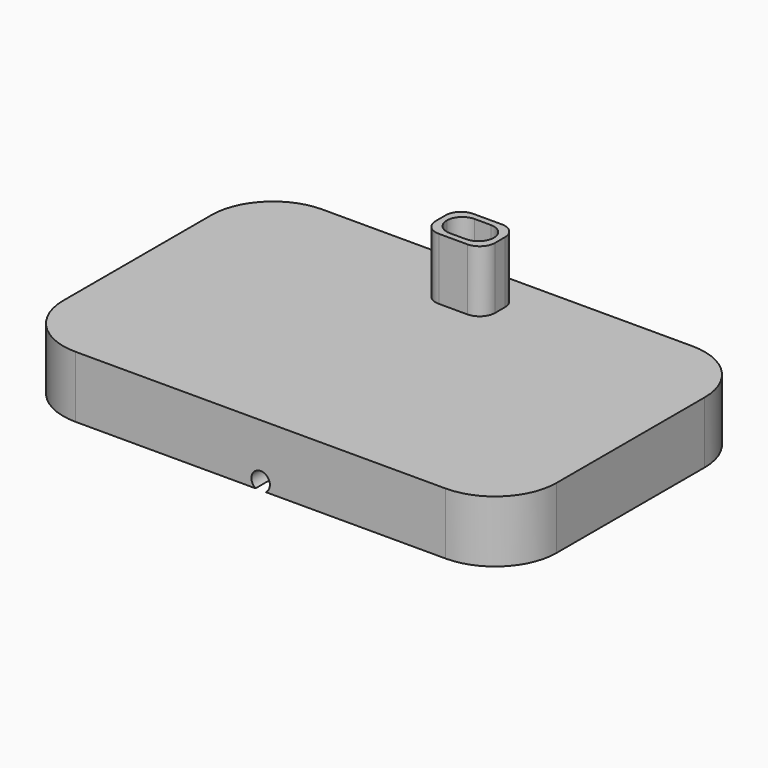
from build123d import *

# Parameters (mm, degrees)
F1_DEPTH = 10
F3_DEPTH = 45
F4_W     = 2.981
F4_H     = 5
F4_W_2   = 1.6583123952
F5_DEPTH = 25
F6_R     = 2.49999
F8_DEPTH = 10
F9_R     = 2.5


# Not quite as in the source:
# - a fillet or chamfer is up to 0.001 mm smaller than in the source, because OpenCascade refuses the exact size
# - ends of sketch curves that miss each other by under 0.0002 mm in the source are joined


with BuildPart() as f1:
    # F0 (on Top) → F1 (new body)
    with BuildSketch(Plane.XY):
        with BuildLine():
            Line((70, 0), (10, 0))
            ThreePointArc((10, 0), (2.9289321881, -2.9289321881), (0, -10))
            Line((0, -10), (0, -40))
            ThreePointArc((0, -40), (2.9289321881, -47.0710678119), (10, -50))
            Line((10, -50), (70, -50))
            ThreePointArc((70, -50), (77.0710678119, -47.0710678119), (80, -40))
            Line((80, -40), (80, -10))
            ThreePointArc((80, -10), (77.0710678119, -2.9289321881), (70, 0))
        make_face()
    extrude(amount=F1_DEPTH)

    # F2 (on face) → F3 (cut)
    with BuildSketch(Plane.XZ.offset(50)):
        with BuildLine():
            ThreePointArc((40.8291561976, 0), (41.3216910184, 0.5406814173), (41.5, 1.25))
            ThreePointArc((41.5, 1.25), (39.2906814173, 2.5716910184), (39.1708438024, 0))
            Line((39.1708438024, 0), (40.8291561976, 0))
        make_face()
    extrude(amount=-F3_DEPTH, mode=Mode.SUBTRACT)

    # F4 (on face) → F5 (cut)
    with BuildSketch(Plane(origin=(0, 0, 0), x_dir=(1, 0, 0), z_dir=(0, 0, -1))):
        with Locations((37.6803438024, 7.5)):
            Rectangle(F4_W, F4_H)
        with Locations((40, 7.5)):
            Rectangle(F4_W_2, F4_H)
        with Locations((42.3196561976, 7.5)):
            Rectangle(F4_W, F4_H)
    extrude(amount=-F5_DEPTH, mode=Mode.SUBTRACT)

    # F6 (radius 2.5 in the source; OpenCascade refuses exactly that, so slightly less here)
    f6_edges = [f1.edges().sort_by_distance(p)[0] for p in [
        (36.189844, -5, 5),
        (43.810156, -5, 5),
        (43.810156, -10, 5),
        (36.189844, -10, 5),
    ]]
    fillet(f6_edges, radius=F6_R)

    # F7 (on face) → F8 (join)
    with BuildSketch(Plane.XY.offset(10)):
        Polygon((35.1898438024, -11), (40, -11), (44.8101561976, -11), (44.8101561976, -4), (35.1898438024, -4), align=None)
        with BuildLine():
            ThreePointArc((38.6898338024, -10), (36.9220739205, -9.2677698819), (36.1898438024, -7.50001))
            ThreePointArc((36.1898438024, -7.50001), (36.9220739205, -5.7322301181), (38.6898338024, -5))
            Line((38.6898338024, -5), (41.3101661976, -5))
            ThreePointArc((41.3101661976, -5), (43.0779260795, -5.7322301181), (43.8101561976, -7.49999))
            ThreePointArc((43.8101561976, -7.49999), (43.0779260795, -9.2677698819), (41.3101661976, -10))
            Line((41.3101661976, -10), (38.6898338024, -10))
        make_face(mode=Mode.SUBTRACT)
    extrude(amount=F8_DEPTH)

    # F9
    f9_edges = [f1.edges().sort_by_distance(p)[0] for p in [
        (44.810156, -4, 15),
        (35.189844, -4, 15),
        (35.189844, -11, 15),
        (44.810156, -11, 15),
    ]]
    fillet(f9_edges, radius=F9_R)


solid = f1.part
